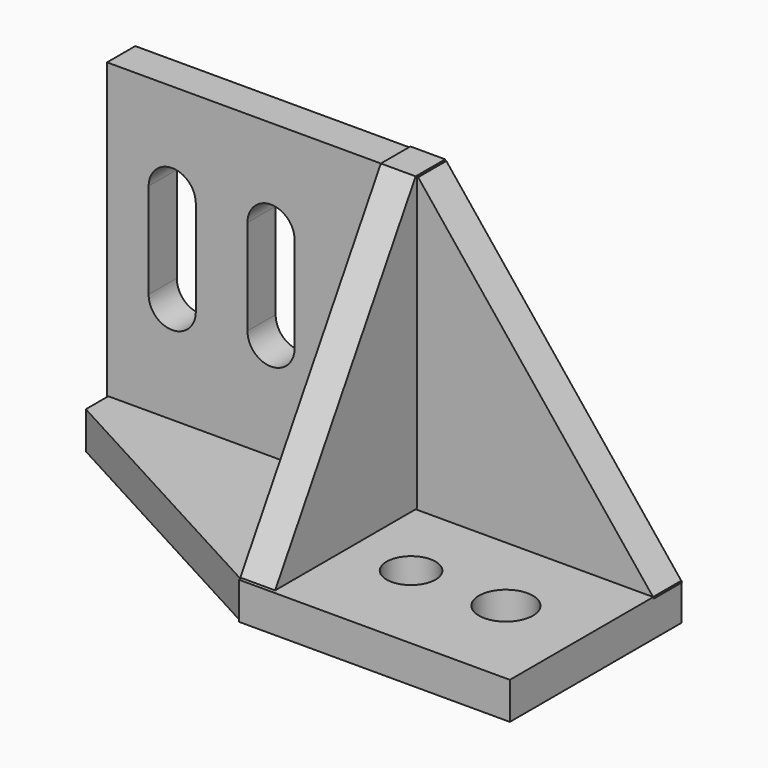
from build123d import *

# Parameters (mm, degrees)
F0_W         = 80.7386888191
F0_H         = 76.366558671
F1_DEPTH     = 9.144
F2_W         = 55.6718036532
F2_H         = 9.6186883748
F3_DEPTH     = 70.358
F4_W         = 9.0357391164
F4_H         = 76.0750807822
F5_DEPTH     = 55.626
F6_SIZE      = 45.72
F7_T1_DEPTH  = 167.084926268
F8_T1_DEPTH  = 193.8162932759
F9_T4_DEPTH  = 127.8865685488
F10_T4_DEPTH = 246.7691481608
F12_DEPTH    = 44.958
F14_DEPTH    = 35.306
F15_R        = 6.35
F15_R_2      = 7.0169538455
F16_DEPTH    = 55.372


# Not quite as in the source:
# - a fillet or chamfer that OpenCascade refuses, or shapes differently, is made with other operations: its cross-section is extruded or revolved along the edge and cut away or added


with BuildPart() as f1:
    # F0 (on Front) → F1 (new body)
    with BuildSketch(Plane.XZ):
        with Locations((-31.0421311297, 2.4775415659)):
            Rectangle(F0_W, F0_H)
        with BuildLine():
            Line((-60.626886785, -8.890000172), (-60.626886785, 15.8854108304))
            ThreePointArc((-60.626886785, 15.8854108304), (-54.5059032738, 22.0063943416), (-48.3849197626, 15.8854108304))
            Line((-48.3849197626, 15.8854108304), (-48.3849197626, -8.890000172))
            ThreePointArc((-48.3849197626, -8.890000172), (-54.5059032738, -15.0109836832), (-60.626886785, -8.890000172))
        make_face(mode=Mode.SUBTRACT)
        with BuildLine():
            Line((-34.9770486355, -8.890000172), (-34.9770486355, 15.8854108304))
            ThreePointArc((-34.9770486355, 15.8854108304), (-28.8560651243, 22.0063943416), (-22.7350816131, 15.8854108304))
            Line((-22.7350816131, 15.8854108304), (-22.7350816131, -8.890000172))
            ThreePointArc((-22.7350816131, -8.890000172), (-28.8560651243, -15.0109836832), (-34.9770486355, -8.890000172))
        make_face(mode=Mode.SUBTRACT)
        Polygon((70.5370530486, -35.7057377696), (9.3272132799, 40.6608209014), (9.3272132799, -35.7057377696), align=None)
    extrude(amount=F1_DEPTH)

    # F2 (on Right) → F3 (join)
    with BuildSketch(Plane.YZ):
        with Locations((-27.8359018266, -40.2236077935)):
            Rectangle(F2_W, F2_H)
    extrude(amount=F3_DEPTH)

    # F4 (on Front) → F5 (join)
    with BuildSketch(Plane.XZ):
        with Locations((4.5178695582, 2.9147546738)):
            Rectangle(F4_W, F4_H)
    extrude(amount=F5_DEPTH)

    # F6
    f6_edges = [f1.edges().sort_by_distance(p)[0] for p in [
        (4.51787, -55.626, 40.952295),
    ]]
    chamfer(f6_edges, length=F6_SIZE)

    # F7: chamfer of 30.48 on 1 edges, made by hand

    # F7_s2 → F7_t1 (cut)
    with BuildSketch(Plane.YZ.offset(-79.0245935758)):
        Polygon((-34.0733853094, 16.7849097555), (-55.626, -35.2477049351), (-55.626, -4.7677049351), align=None)
    extrude(amount=F7_T1_DEPTH, mode=Mode.SUBTRACT)

    # F8: chamfer of 35.56 on 1 edges, made by hand

    # F8_s2 → F8_t1 (cut)
    with BuildSketch(Plane.YZ.offset(-92.3902770798)):
        Polygon((-8.9286681704, 41.9296268945), (-47.6816081643, -16.0682464206), (-34.0733853094, 16.7849097555), align=None)
    extrude(amount=F8_T1_DEPTH, mode=Mode.SUBTRACT)

    # F9: chamfer of 22.86 on 1 edges, made by hand


with BuildPart() as f9_tool2:
    # F9_s3 → F9_t4 (new body)
    with BuildSketch(Plane.YZ.offset(-59.4254147162)):
        Polygon((-34.9812726375, 2.9391489166), (-56.4297514282, -37.1881325338), (-47.6816081643, -16.0682464206), align=None)
    extrude(amount=F9_T4_DEPTH)

    split(bisect_by=Plane.XY.offset(-35.4142636061), keep=Keep.TOP)


with BuildPart() as f1_1:
    add(f1.part)

    # F9_t1: cut F9_tool2
    add(f9_tool2.part, mode=Mode.SUBTRACT)

    # F10: chamfer of 45.72 on 1 edges, made by hand


with BuildPart() as f10_tool2:
    # F10_s3 → F10_t4 (new body)
    with BuildSketch(Plane.YZ.offset(-118.8667045222)):
        Polygon((-56.5335314452, -37.3822912894), (-9.5806015838, 40.9539395911), (-34.9812726375, 2.9391489166), align=None)
    extrude(amount=F10_T4_DEPTH)

    split(bisect_by=Plane.XY.offset(-35.1227857172), keep=Keep.TOP)


with BuildPart() as f1_2:
    add(f1_1.part)

    # F10_t1: cut F10_tool2
    add(f10_tool2.part, mode=Mode.SUBTRACT)

    # F11 (on Top) → F12 (join)
    with BuildSketch(Plane.XY):
        Polygon((-70.8285272121, -16.7598351836), (0, -55.2345886827), (0, -9.472951293), (-70.8285272121, -9.472951293), align=None)
    extrude(amount=-F12_DEPTH)

    # F13 (on Top) → F14 (cut)
    with BuildSketch(Plane.XY):
        Polygon((0, -9.1814752668), (-71.4114755392, -9.1814752668), (-71.4114755392, -16.4683610201), (0, -55.8175444603), align=None)
    extrude(amount=-F14_DEPTH, mode=Mode.SUBTRACT)

    # F15 (on Top) → F16 (cut)
    with BuildSketch(Plane.XY):
        with Locations((24.775644736, -30.7506565005)):
            Circle(F15_R)
        with Locations((49.3974882285, -30.7506565005)):
            Circle(F15_R_2)
    extrude(amount=-F16_DEPTH, mode=Mode.SUBTRACT)


solid = f1_2.part
